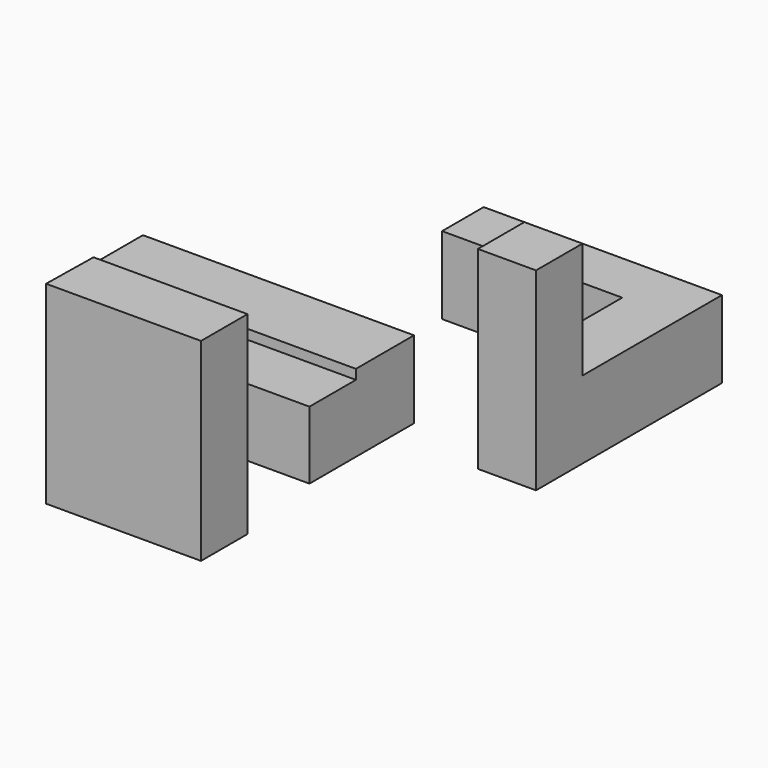
from build123d import *

# Parameters (mm, degrees)
F3_DEPTH = 800
F4_DEPTH = 2000
F0_W     = 600
F0_H     = 600
F5_DEPTH = 2000
F6_DEPTH = 800
F0_W_2   = 1400.595679329
F7_DEPTH = 700


# Not quite as in the source:
# - the program builds the solid bodies; features that only make, move or delete a surface that nothing else refers to are left out


with BuildPart() as f3:
    # F0 (on Top) → F3 (new body)
    with BuildSketch(Plane.XY):
        Polygon((-1399.404320671, 600), (-1399.404320671, 0), (0, 0), (0, -150), (1400.595679329, -150), (1400.595679329, 600), align=None)
    extrude(amount=F3_DEPTH)

    # F0 (on Top) → F7 (join)
    with BuildSketch(Plane.XY):
        with Locations((700.2978396645, -450)):
            Rectangle(F0_W_2, F0_H)
    extrude(amount=F7_DEPTH)


with BuildPart() as f4:
    # F0 (on Top) → F4 (new body)
    with BuildSketch(Plane.XY):
        Polygon((1560.595679329, -1750), (-29.3436430529, -1750), (-39.404320671, -2350), (1560.595679329, -2350), align=None)
    extrude(amount=F4_DEPTH)


with BuildPart() as f5:
    # F0 (on Top) → F5 (new body, through all)
    with BuildSketch(Plane.XY):
        with Locations((2600.595679329, 600)):
            Rectangle(F0_W, F0_H)
    extrude(amount=F5_DEPTH)

    # F0 (on Top) → F6 (join, through all)
    with BuildSketch(Plane.XY):
        Polygon((490.595679329, 2700), (440.3408169746, 2700), (440.3408169746, 2162.5823974609), (2300.595679329, 2162.5823974609), (2300.595679329, 900), (2900.595679329, 900), (2900.595679329, 2700), (2150.595679329, 2700), align=None)
    extrude(amount=F6_DEPTH)


solid = Compound([f3.part, f4.part, f5.part])
